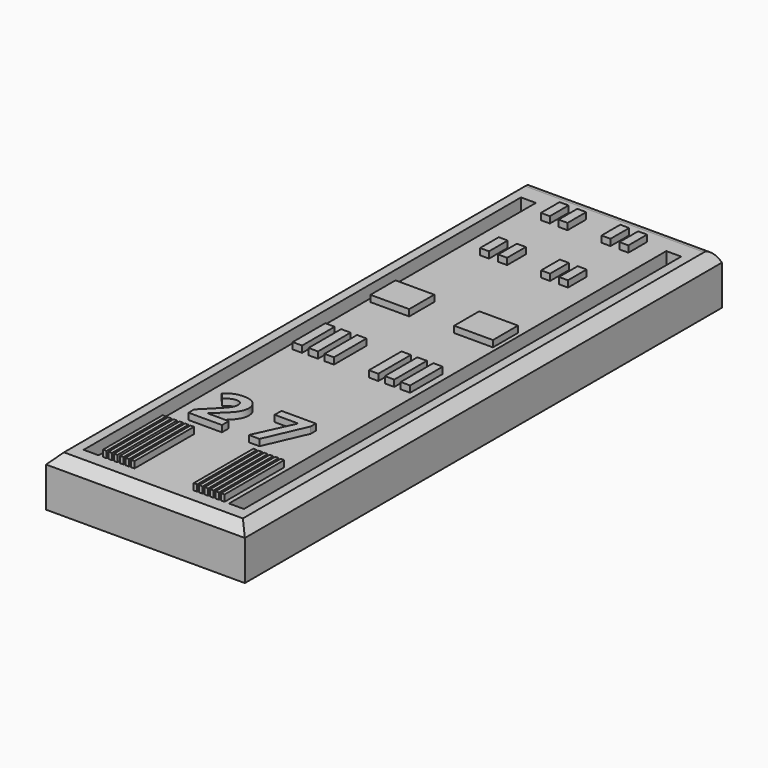
from build123d import *

# Parameters (mm, degrees)
F0_W         = 7.62
F0_H         = 279.4
F1_DEPTH     = 25.4
F4_W         = 1.778
F4_H         = 38.1
F4_W_2       = 4.826
F4_H_2       = 20.828
F4_W_3       = 19.812
F4_H_3       = 16.002
F4_W_4       = 4.572
F4_H_4       = 11.938
F4_TEXT_SIZE = 34.2266731882
F5_DEPTH     = 3.302
F6_SIZE      = 5.08
F7_SIZE      = 5.08
F8_R         = 5.08


# Not quite as in the source:
# - the program builds the solid bodies; features that only make, move or delete a surface that nothing else refers to are left out
# - Text() gives the source's letters only with a copy of the font that has no kerning and outlines rounded to 1/6400 em; it was checked with that copy


with BuildPart() as f1:
    # F0 (on Top) → F1 (new body)
    with BuildSketch(Plane.XY):
        Polygon((50.8, 152.4), (0, 152.4), (-50.8, 152.4), (-50.8, -152.4), (0, -152.4), (50.8, -152.4), align=None)
        with Locations((-37.1395085478, -1.0004743814)):
            Rectangle(F0_W, F0_H, mode=Mode.SUBTRACT)
        with Locations((37.1395085478, -1.0004743814)):
            Rectangle(F0_W, F0_H, mode=Mode.SUBTRACT)
    extrude(amount=F1_DEPTH)

    # F4 (on face) → F5 (join)
    with BuildSketch(Plane.XY.offset(25.4)):
        with Locations((-30.1545085478, -121.6504743814)):
            Rectangle(F4_W, F4_H)
        with Locations((-27.3605085478, -121.6504743814)):
            Rectangle(F4_W, F4_H)
        with Locations((-24.5665085478, -121.6504743814)):
            Rectangle(F4_W, F4_H)
        with Locations((-21.5114120682, -121.6504743814)):
            Rectangle(F4_W, F4_H)
        with Locations((-18.7174120682, -121.6504743814)):
            Rectangle(F4_W, F4_H)
        Polygon((-15.0344120682, -102.6004743814), (-16.8124120682, -102.6004743814), (-16.8124120682, -140.7004743814), (-15.0344120682, -140.646442771), align=None)
        with Locations((30.1545085478, -121.6504743814)):
            Rectangle(F4_W, F4_H)
        with Locations((27.3605085478, -121.6504743814)):
            Rectangle(F4_W, F4_H)
        with Locations((24.5665085478, -121.6504743814)):
            Rectangle(F4_W, F4_H)
        with Locations((21.7725085478, -121.6504743814)):
            Rectangle(F4_W, F4_H)
        with Locations((18.9785085478, -121.6504743814)):
            Rectangle(F4_W, F4_H)
        with Locations((16.1845085478, -121.6504743814)):
            Rectangle(F4_W, F4_H)
        with Locations((-27.6145085478, -10.414)):
            Rectangle(F4_W_2, F4_H_2)
        with Locations((-19.4865085478, -10.414)):
            Rectangle(F4_W_2, F4_H_2)
        with Locations((-11.3585085478, -10.414)):
            Rectangle(F4_W_2, F4_H_2)
        with Locations((27.6145085478, -10.414)):
            Rectangle(F4_W_2, F4_H_2)
        with Locations((19.4865085478, -10.414)):
            Rectangle(F4_W_2, F4_H_2)
        with Locations((11.3585085478, -10.414)):
            Rectangle(F4_W_2, F4_H_2)
        with Locations((-21.3915085478, 38.4643248597)):
            Rectangle(F4_W_3, F4_H_3)
        with Locations((21.3915085478, 38.4643248597)):
            Rectangle(F4_W_3, F4_H_3)
        with Locations((-20.1215085478, 95.3717128816)):
            Rectangle(F4_W_4, F4_H_4)
        with Locations((-10.9775085478, 95.4987108707)):
            Rectangle(F4_W_4, F4_H_4)
        with Locations((10.9775085478, 95.4987108707)):
            Rectangle(F4_W_4, F4_H_4)
        with Locations((20.1215085478, 95.4987108707)):
            Rectangle(F4_W_4, F4_H_4)
        with Locations((-10.9775085478, 134.1067105532)):
            Rectangle(F4_W_4, F4_H_4)
        with Locations((-20.1215085478, 134.2337085423)):
            Rectangle(F4_W_4, F4_H_4)
        with Locations((10.9775085478, 134.1067105532)):
            Rectangle(F4_W_4, F4_H_4)
        with Locations((20.1215085478, 134.1067105532)):
            Rectangle(F4_W_4, F4_H_4)
        with Locations((-25.7159691393, -94.4607533612)):
            Text('2 7', F4_TEXT_SIZE, font='Open Sans', font_style=FontStyle.BOLD, text_align=(TextAlign.LEFT, TextAlign.BOTTOM))
    extrude(amount=F5_DEPTH)

    # F6
    f6_edges = [f1.edges().sort_by_distance(p)[0] for p in [
        (50.8, 0, 25.4),
        (-50.8, 0, 25.4),
    ]]
    chamfer(f6_edges, length=F6_SIZE)

    # F7
    f7_edges = [f1.edges().sort_by_distance(p)[0] for p in [
        (0, -152.4, 25.4),
    ]]
    chamfer(f7_edges, length=F7_SIZE)

    # F8
    f8_edges = [f1.edges().sort_by_distance(p)[0] for p in [
        (0, 152.4, 25.4),
    ]]
    fillet(f8_edges, radius=F8_R)


solid = f1.part
